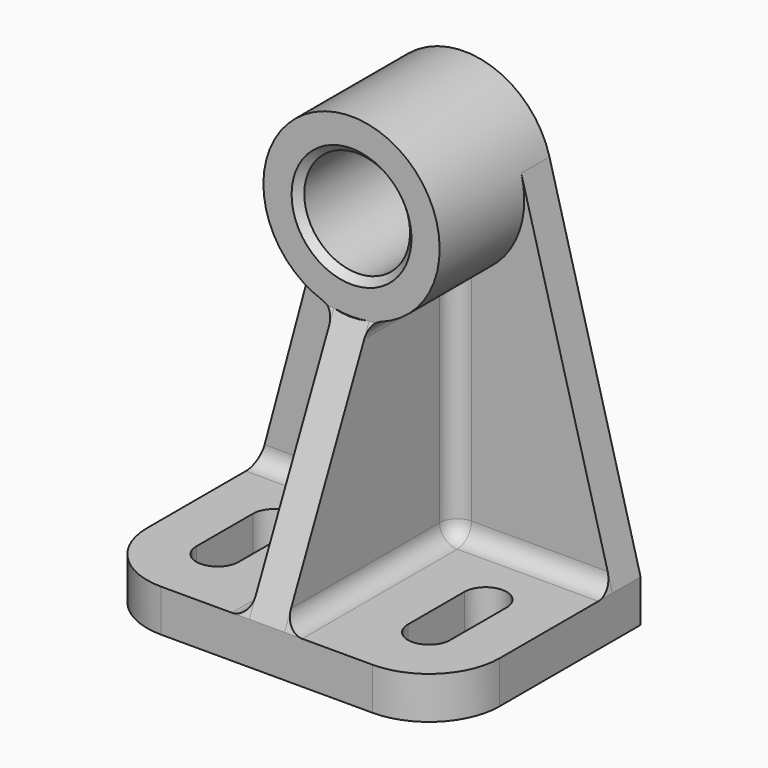
from build123d import *

# Parameters (mm, degrees)
F1_DEPTH      = 304.8
F3_DEPTH      = 254
F2_R          = 381
F4_DEPTH      = 1016
F5_SIZE       = 50.8
F7_DEPTH      = 1524
F9_DEPTH      = 279.4
F10_T1_DEPTH  = 1002.6252375466
F10_S5_W      = 129.54
F10_S5_H      = 129.54
F10_T6_DEPTH  = 129.54
F10_S11_W     = 129.54
F10_S11_H     = 129.54
F10_T12_DEPTH = 129.54
F10_T18_DEPTH = 1333.5
F10_T23_DEPTH = 1714.5
F10_T28_DEPTH = 1854.5825321713
F10_S29_R     = 635
F10_T30_DEPTH = 933
F10_T34_DEPTH = 1854.5825321713
F10_S35_R     = 635
F10_T36_DEPTH = 933
F10_T40_DEPTH = 1333.5
F10_T45_DEPTH = 1714.5
F10_T50_DEPTH = 1243.2504750931
F10_T55_DEPTH = 1243.2504750931


# Not quite as in the source:
# - a fillet or chamfer that OpenCascade refuses, or shapes differently, is made with other operations: its cross-section is extruded or revolved along the edge and cut away or added


with BuildPart() as f1:
    # F0 (on Top) → F1 (new body)
    with BuildSketch(Plane.XY):
        with BuildLine():
            Line((0, 0), (-1270, 0))
            Line((-1270, 0), (-1270, -1270))
            ThreePointArc((-1270, -1270), (-1121.2102448428, -1629.2102448428), (-762, -1778))
            Line((-762, -1778), (762, -1778))
            ThreePointArc((762, -1778), (1121.2102448428, -1629.2102448428), (1270, -1270))
            Line((1270, -1270), (1270, 0))
            Line((1270, 0), (0, 0))
        make_face()
        with BuildLine():
            ThreePointArc((-609.6, -1270.0000219048), (-762, -1422.4), (-914.4, -1270.0000219048))
            Line((-914.4, -1270.0000219048), (-914.4, -762.0000219048))
            ThreePointArc((-914.4, -762.0000219048), (-762, -609.6000219048), (-609.6, -762.0000219048))
            Line((-609.6, -762.0000219048), (-609.6, -1270.0000219048))
        make_face(mode=Mode.SUBTRACT)
        with BuildLine():
            ThreePointArc((609.6, -762.0000219048), (762, -609.6000219048), (914.4, -762.0000219048))
            Line((914.4, -762.0000219048), (914.4, -1270.0000219048))
            ThreePointArc((914.4, -1270.0000219048), (762, -1422.4), (609.6, -1270.0000219048))
            Line((609.6, -1270.0000219048), (609.6, -762.0000219048))
        make_face(mode=Mode.SUBTRACT)
    extrude(amount=F1_DEPTH)

    # F2 (on face) → F3 (join)
    with BuildSketch(Plane(origin=(0, 0, 0), x_dir=(-1, 0, 0), z_dir=(0, 1, 0))):
        with BuildLine():
            Line((-613.3628996936, 2755.4030204783), (-1270, 304.8))
            Line((-1270, 304.8), (1270, 304.8))
            Line((1270, 304.8), (613.3628996936, 2755.4030204783))
            ThreePointArc((613.3628996936, 2755.4030204783), (629.5674869724, 2673.937058898), (635, 2591.0529268382))
            ThreePointArc((635, 2591.0529268382), (-82.8841320597, 1961.4854398659), (-613.3628996936, 2755.4030204783))
        make_face()
    extrude(amount=-F3_DEPTH)

    # F2 (on face) → F4 (join)
    with BuildSketch(Plane(origin=(0, 0, 0), x_dir=(-1, 0, 0), z_dir=(0, 1, 0))):
        with BuildLine():
            ThreePointArc((613.3628996936, 2755.4030204783), (0, 3226.0529268382), (-613.3628996936, 2755.4030204783))
            ThreePointArc((-613.3628996936, 2755.4030204783), (-82.8841320597, 1961.4854398659), (635, 2591.0529268382))
            ThreePointArc((635, 2591.0529268382), (629.5674869724, 2673.937058898), (613.3628996936, 2755.4030204783))
        make_face()
        with Locations((0, 2591.0529268382)):
            Circle(F2_R, mode=Mode.SUBTRACT)
    extrude(amount=-F4_DEPTH)

    # F5
    f5_edges = [f1.edges().sort_by_distance(p)[0] for p in [
        (381, -1016, 2591.052927),
    ]]
    chamfer(f5_edges, length=F5_SIZE)

    # F6 (on face) → F7 (join)
    with BuildSketch(Plane.XZ.offset(254)):
        with BuildLine():
            Line((-127, 1968.8825321713), (-127, 304.8))
            Line((-127, 304.8), (127, 304.8))
            Line((127, 304.8), (127, 1968.8825321713))
            ThreePointArc((127, 1968.8825321713), (0, 1956.0529268382), (-127, 1968.8825321713))
        make_face()
    extrude(amount=F7_DEPTH)

    # F8 (on face) → F9 (cut)
    with BuildSketch(Plane.YZ.offset(127)):
        Polygon((-1778, 1968.8825321713), (-1778, 304.8), (-1016, 1968.8825321713), align=None)
    extrude(amount=-F9_DEPTH, mode=Mode.SUBTRACT)

    # F10: fillet of radius 127 on 8 edges, made by hand

    # F10_s2 → F10_t1 (join)
    with BuildSketch(Plane.XZ.offset(13.3747624534)):
        with BuildLine():
            ThreePointArc((127, 1872.6324371527), (150.3049342222, 1945.9559213398), (211.6666666667, 1992.3691854336))
            ThreePointArc((211.6666666667, 1992.3691854336), (169.7400468309, 1979.1597037169), (127, 1968.8825321713))
            Line((127, 1968.8825321713), (127, 1872.6324371527))
        make_face()
        with BuildLine():
            ThreePointArc((-127, 1872.6324371527), (-150.3049342222, 1945.9559213398), (-211.6666666667, 1992.3691854336))
            ThreePointArc((-211.6666666667, 1992.3691854336), (-169.7400468309, 1979.1597037169), (-127, 1968.8825321713))
            Line((-127, 1968.8825321713), (-127, 1872.6324371527))
        make_face()
    extrude(amount=F10_T1_DEPTH)


with BuildPart() as f10_tool4:
    # F10_s5 → F10_t6 (new body)
    with BuildSketch(Plane.YZ.offset(-254)):
        with Locations((-316.23, 367.03)):
            Rectangle(F10_S5_W, F10_S5_H)
    extrude(amount=F10_T6_DEPTH)

    # F10_s7 → F10_t8 (revolve, cut)
    with BuildSketch(Plane(origin=(-254, -381, 431.8), x_dir=(0, -0.7071067812, 0.7071067812), z_dir=(0, 0.7071067812, 0.7071067812))):
        with BuildLine():
            ThreePointArc((0, -127), (127, 0), (0, 127))
            Line((0, 127), (0, -127))
        make_face()
    revolve(axis=Axis((-254, -381, 431.8), (1, 0, 0)), mode=Mode.SUBTRACT)


with BuildPart() as f1_1:
    add(f1.part)

    # F10_t3: union F10_tool4
    add(f10_tool4.part)


with BuildPart() as f10_tool10:
    # F10_s11 → F10_t12 (new body)
    with BuildSketch(Plane.XY.offset(431.8)):
        with Locations((189.23, -316.23)):
            Rectangle(F10_S11_W, F10_S11_H)
    extrude(amount=-F10_T12_DEPTH)

    # F10_s13 → F10_t14 (revolve, cut)
    with BuildSketch(Plane(origin=(254, -381, 431.8), x_dir=(0.7071067812, -0.7071067812, 0), z_dir=(0.7071067812, 0.7071067812, 0))):
        with BuildLine():
            ThreePointArc((0, -127), (127, 0), (0, 127))
            Line((0, 127), (0, -127))
        make_face()
    revolve(axis=Axis((254, -381, 431.8), (0, 0, -1)), mode=Mode.SUBTRACT)


with BuildPart() as f1_2:
    add(f1_1.part)

    # F10_t9: union F10_tool10
    add(f10_tool10.part)


with BuildPart() as f10_tool16:
    # F10_s17 → F10_t18 (new body)
    with BuildSketch(Plane.YZ.offset(-254)):
        with BuildLine():
            ThreePointArc((-381, 304.8), (-291.1974387893, 341.9974387893), (-254, 431.8))
            Line((-254, 431.8), (-254, 304.8))
            Line((-254, 304.8), (-381, 304.8))
        make_face()
    extrude(amount=-F10_T18_DEPTH)

    split(bisect_by=Plane(origin=(-1261.1261314031, 0, 337.9177284633), x_dir=(0, 1, 0), z_dir=(0.9659258263, 0, -0.2588190451)), keep=Keep.TOP)


with BuildPart() as f1_3:
    add(f1_2.part)

    # F10_t15: union F10_tool16
    add(f10_tool16.part)


with BuildPart() as f10_tool21:
    # F10_s22 → F10_t23 (new body)
    with BuildSketch(Plane.XZ.offset(381)):
        with BuildLine():
            ThreePointArc((-127, 431.8), (-164.1974387893, 341.9974387893), (-254, 304.8))
            Line((-254, 304.8), (-127, 304.8))
            Line((-127, 304.8), (-127, 431.8))
        make_face()
    extrude(amount=F10_T23_DEPTH)

    split(bisect_by=Plane(origin=(0, -1585.1865820182, 725.8727569971), x_dir=(1, 0, 0), z_dir=(0, 0.9092105607, -0.4163365902)), keep=Keep.TOP)


with BuildPart() as f1_4:
    add(f1_3.part)

    # F10_t20: union F10_tool21
    add(f10_tool21.part)


with BuildPart() as f10_tool26:
    # F10_s27 → F10_t28 (new body)
    with BuildSketch(Plane.XY.offset(2286.3825321713)):
        with BuildLine():
            ThreePointArc((-127, -381), (-164.1974387893, -291.1974387893), (-254, -254))
            Line((-254, -254), (-127, -254))
            Line((-127, -254), (-127, -381))
        make_face()
    extrude(amount=-F10_T28_DEPTH)

    # F10_s29 → F10_t30 (cut, symmetric)
    with BuildSketch(Plane.XZ.offset(317.5)):
        with Locations((0, 2591.0529268382)):
            Circle(F10_S29_R)
    extrude(amount=F10_T30_DEPTH, both=True, mode=Mode.SUBTRACT)


with BuildPart() as f1_5:
    add(f1_4.part)

    # F10_t25: union F10_tool26
    add(f10_tool26.part)


with BuildPart() as f10_tool32:
    # F10_s33 → F10_t34 (new body)
    with BuildSketch(Plane.XY.offset(431.8)):
        with BuildLine():
            ThreePointArc((254, -254), (164.1974387893, -291.1974387893), (127, -381))
            Line((127, -381), (127, -254))
            Line((127, -254), (254, -254))
        make_face()
    extrude(amount=F10_T34_DEPTH)

    # F10_s35 → F10_t36 (cut, symmetric)
    with BuildSketch(Plane.XZ.offset(317.5)):
        with Locations((0, 2591.0529268382)):
            Circle(F10_S35_R)
    extrude(amount=F10_T36_DEPTH, both=True, mode=Mode.SUBTRACT)


with BuildPart() as f1_6:
    add(f1_5.part)

    # F10_t31: union F10_tool32
    add(f10_tool32.part)


with BuildPart() as f10_tool38:
    # F10_s39 → F10_t40 (new body)
    with BuildSketch(Plane.YZ.offset(1587.5)):
        with BuildLine():
            ThreePointArc((-381, 304.8), (-291.1974387893, 341.9974387893), (-254, 431.8))
            Line((-254, 431.8), (-254, 304.8))
            Line((-254, 304.8), (-381, 304.8))
        make_face()
    extrude(amount=-F10_T40_DEPTH)

    split(bisect_by=Plane(origin=(1261.1261314031, 0, 337.9177284633), x_dir=(0, 1, 0), z_dir=(-0.9659258263, 0, -0.2588190451)), keep=Keep.TOP)


with BuildPart() as f1_7:
    add(f1_6.part)

    # F10_t37: union F10_tool38
    add(f10_tool38.part)


with BuildPart() as f10_tool43:
    # F10_s44 → F10_t45 (new body)
    with BuildSketch(Plane.XZ.offset(381)):
        with BuildLine():
            ThreePointArc((254, 304.8), (164.1974387893, 341.9974387893), (127, 431.8))
            Line((127, 431.8), (127, 304.8))
            Line((127, 304.8), (254, 304.8))
        make_face()
    extrude(amount=F10_T45_DEPTH)

    split(bisect_by=Plane(origin=(0, -1585.1865820182, 725.8727569971), x_dir=(1, 0, 0), z_dir=(0, 0.9092105607, -0.4163365902)), keep=Keep.TOP)


with BuildPart() as f1_8:
    add(f1_7.part)

    # F10_t42: union F10_tool43
    add(f10_tool43.part)


with BuildPart() as f10_tool48:
    # F10_s49 → F10_t50 (new body)
    with BuildSketch(Plane.XZ.offset(13.3747624534)):
        with BuildLine():
            ThreePointArc((127, 1872.6324371527), (150.3049342222, 1945.9559213398), (211.6666666667, 1992.3691854336))
            ThreePointArc((211.6666666667, 1992.3691854336), (169.7400468309, 1979.1597037169), (127, 1968.8825321713))
            Line((127, 1968.8825321713), (127, 1872.6324371527))
        make_face()
    extrude(amount=F10_T50_DEPTH)

    split(bisect_by=Plane(origin=(0, -1585.1865820182, 725.8727569971), x_dir=(1, 0, 0), z_dir=(0, 0.9092105607, -0.4163365902)), keep=Keep.TOP)


with BuildPart() as f1_9:
    add(f1_8.part)

    # F10_t47: union F10_tool48
    add(f10_tool48.part)


with BuildPart() as f10_tool53:
    # F10_s54 → F10_t55 (new body)
    with BuildSketch(Plane.XZ.offset(13.3747624535)):
        with BuildLine():
            ThreePointArc((-127, 1872.6324371527), (-150.3049342222, 1945.9559213398), (-211.6666666667, 1992.3691854336))
            ThreePointArc((-211.6666666667, 1992.3691854336), (-169.7400468309, 1979.1597037169), (-127, 1968.8825321713))
            Line((-127, 1968.8825321713), (-127, 1872.6324371527))
        make_face()
    extrude(amount=F10_T55_DEPTH)

    split(bisect_by=Plane(origin=(0, -1585.1865820182, 725.8727569971), x_dir=(1, 0, 0), z_dir=(0, 0.9092105607, -0.4163365902)), keep=Keep.TOP)


with BuildPart() as f1_10:
    add(f1_9.part)

    # F10_t52: union F10_tool53
    add(f10_tool53.part)


solid = f1_10.part
